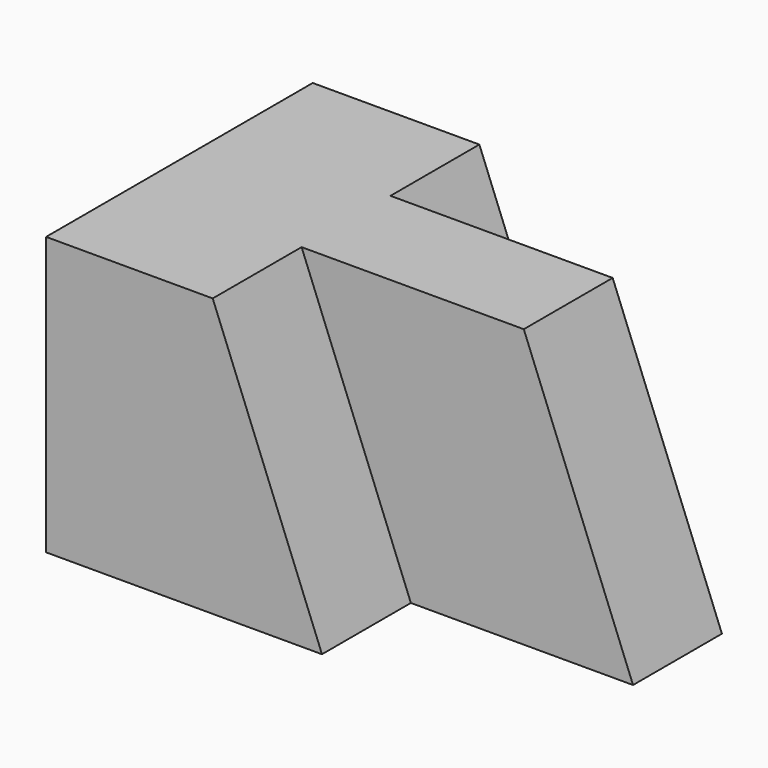
from build123d import *

# Parameters (mm, degrees)
F1_DEPTH = 25.4
F3_DEPTH = 38.1
F5_DEPTH = 12.7
F6_DEPTH = 12.7
F8_DEPTH = 12.7


# Not quite as in the source:
# - a length typed as a fraction of an inch, garbled in the dataset ("3 / 203.2 mm" for 3/8 in), is restored


with BuildPart() as f1:
    # F0 (on Front) → F1 (new body)
    with BuildSketch(Plane.XZ):
        Polygon((57.15, 31.7493037554), (0, 31.7493037554), (0, 0), (56.9397357658, 0), align=None)
    extrude(amount=F1_DEPTH)

    # F2 (on face) → F3 (cut)
    with BuildSketch(Plane.XZ.offset(25.4)):
        Polygon((44.45, 31.7493037554), (56.9397357658, 0), (57.15, 31.7493037554), align=None)
    extrude(amount=-F3_DEPTH, mode=Mode.SUBTRACT)

    # F4 (on face) → F5 (cut)
    with BuildSketch(Plane.XZ.offset(25.4)):
        Polygon((44.45, 31.7493037554), (19.05, 31.7493037554), (31.5397357658, 0), (56.9397357658, 0), align=None)
    extrude(amount=-F5_DEPTH, mode=Mode.SUBTRACT)

    # F6 (add): a face of the model
    f6_faces = [f1.faces().sort_by_distance(p)[0] for p in [
        (25.4756467057, 0, 15.2228100654),
    ]]
    extrude(f6_faces, amount=F6_DEPTH)

    # F7 (on face) → F8 (cut)
    with BuildSketch(Plane(origin=(0, 12.7, 0), x_dir=(-1, 0, 0), z_dir=(0, 1, 0))):
        Polygon((-56.9397357658, 0), (-31.5397357658, 0), (-19.05, 31.7493037554), (-44.45, 31.7493037554), align=None)
    extrude(amount=-F8_DEPTH, mode=Mode.SUBTRACT)


solid = f1.part
